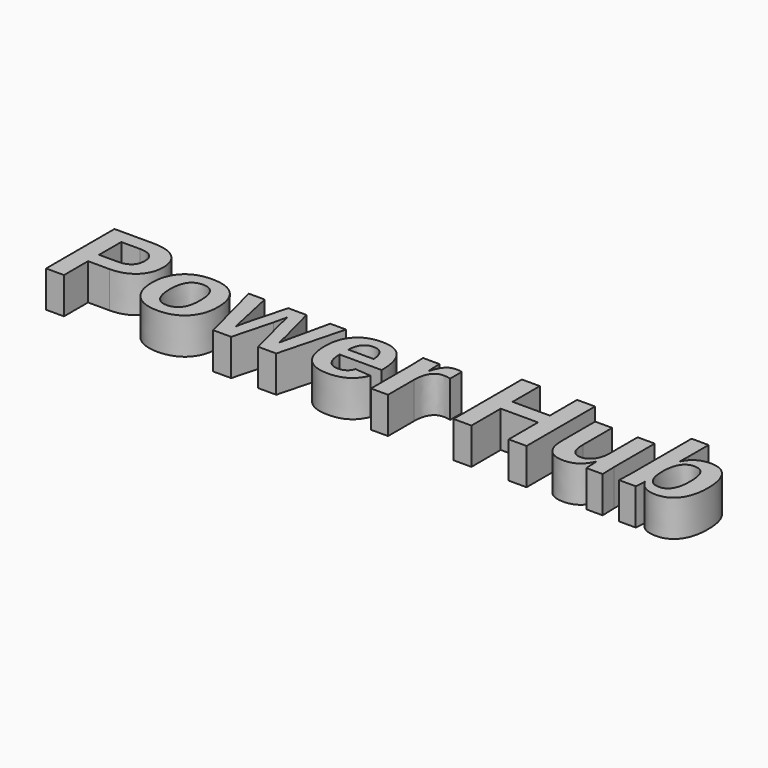
from build123d import *

# Parameters (mm, degrees)
F0_TEXT_SIZE = 6.8326522726
F1_DEPTH     = 2


# Not quite as in the source:
# - a feature names something its author has since deleted; it is built from what else it names
# - Text() gives the source's letters only with a copy of the font that has no kerning and outlines rounded to 1/6400 em; it was checked with that copy


with BuildPart() as f1:
    # F0 (on Top) → F1 (new body)
    with BuildSketch(Plane.XY):
        with Locations((12.2161991894, -2.8566406108)):
            Text('Power Hub', F0_TEXT_SIZE, font='Arimo', font_style=FontStyle.BOLD, text_align=(TextAlign.LEFT, TextAlign.BOTTOM))
    extrude(amount=F1_DEPTH)


solid = f1.part
